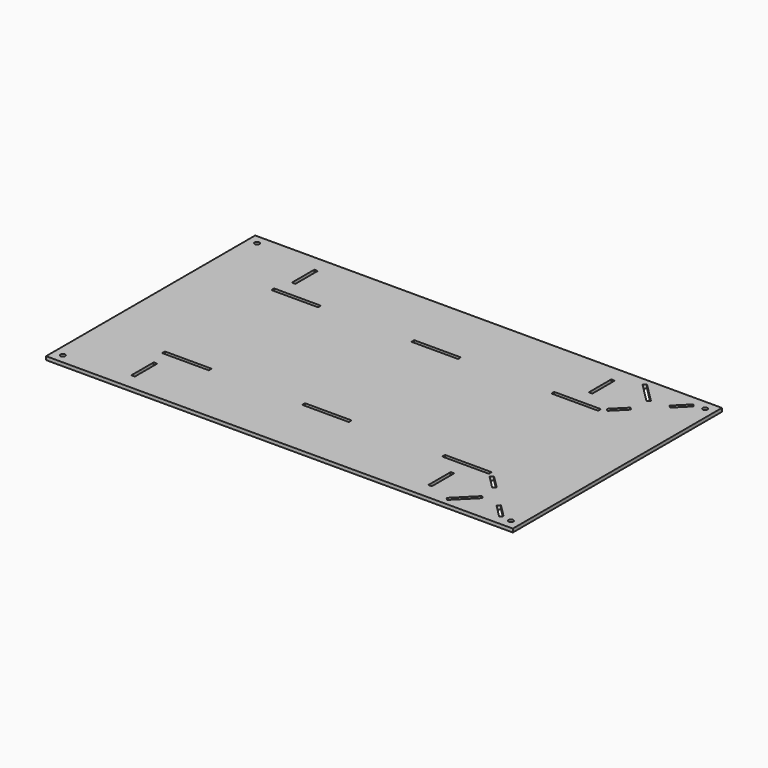
from build123d import *

# Parameters (mm, degrees)
F0_W     = 3.75
F0_H     = 30
F0_W_2   = 50
F0_H_2   = 3.75
F1_DEPTH = 3.75
F3_D     = 5
F5_DEPTH = 3.75


# Not quite as in the source:
# - a feature names something its author has since deleted; it is built from what else it names


with BuildPart() as f1:
    # F0 (on Top) → F1 (new body)
    with BuildSketch(Plane.XY):
        Polygon((-37.9051826894, 0), (12.0948173106, 0), (462.0948173106, 0), (462.0948173106, 280), (62.0948173106, 280), (-37.9051826894, 280), align=None)
        with Locations((41.3065613726, 32.5)):
            Rectangle(F0_W, F0_H, mode=Mode.SUBTRACT)
        with Locations((59.4315613726, 66.875)):
            Rectangle(F0_W_2, F0_H_2, mode=Mode.SUBTRACT)
        with Locations((209.4315613726, 66.875)):
            Rectangle(F0_W_2, F0_H_2, mode=Mode.SUBTRACT)
        with Locations((359.4315613726, 32.5)):
            Rectangle(F0_W, F0_H, mode=Mode.SUBTRACT)
        with Locations((359.4315613726, 66.875)):
            Rectangle(F0_W_2, F0_H_2, mode=Mode.SUBTRACT)
        with Locations((59.4315613726, 213.125)):
            Rectangle(F0_W_2, F0_H_2, mode=Mode.SUBTRACT)
        with Locations((41.3065613726, 247.5)):
            Rectangle(F0_W, F0_H, mode=Mode.SUBTRACT)
        with Locations((209.4315613726, 213.125)):
            Rectangle(F0_W_2, F0_H_2, mode=Mode.SUBTRACT)
        with Locations((359.4315613726, 213.125)):
            Rectangle(F0_W_2, F0_H_2, mode=Mode.SUBTRACT)
        with Locations((359.4315613726, 247.5)):
            Rectangle(F0_W, F0_H, mode=Mode.SUBTRACT)
    extrude(amount=F1_DEPTH)

    # F3 (through all)
    with Locations(Plane.XY.offset(3.75)):
        with Locations((-27.9051826894, 10), (-27.9051826894, 270), (452.0948173106, 10), (452.0948173106, 270)):
            Hole(F3_D / 2)

    # F4 (on face) → F5 (cut)
    with BuildSketch(Plane.XY.offset(3.75)):
        Polygon((442.083211802, 267.3483495706), (439.4315613726, 270), (425.2894257488, 255.8578643763), (427.9410761783, 253.2062139468), align=None)
        Polygon((402.1092280247, 232.6776666521), (387.9670924009, 218.5355310284), (390.6187428304, 215.8838805989), (404.7608784541, 230.0260162227), align=None)
        Polygon((386.740880854, 273.8778619764), (384.0892304246, 271.2262115469), (405.3024338602, 250.0130081113), (407.9540842896, 252.6646585408), align=None)
        Polygon((387.9670924009, 61.4644689716), (402.1092280247, 47.3223333479), (404.7608784541, 49.9739837773), (390.6187428304, 64.1161194011), align=None)
        Polygon((405.3024338602, 29.9869918887), (384.0892304246, 8.7737884531), (386.740880854, 6.1221380236), (407.9540842896, 27.3353414592), align=None)
        Polygon((427.9410761783, 26.7937860532), (425.2894257488, 24.1421356237), (439.4315613726, 10), (442.083211802, 12.6516504294), align=None)
    extrude(amount=-F5_DEPTH, mode=Mode.SUBTRACT)


solid = f1.part
